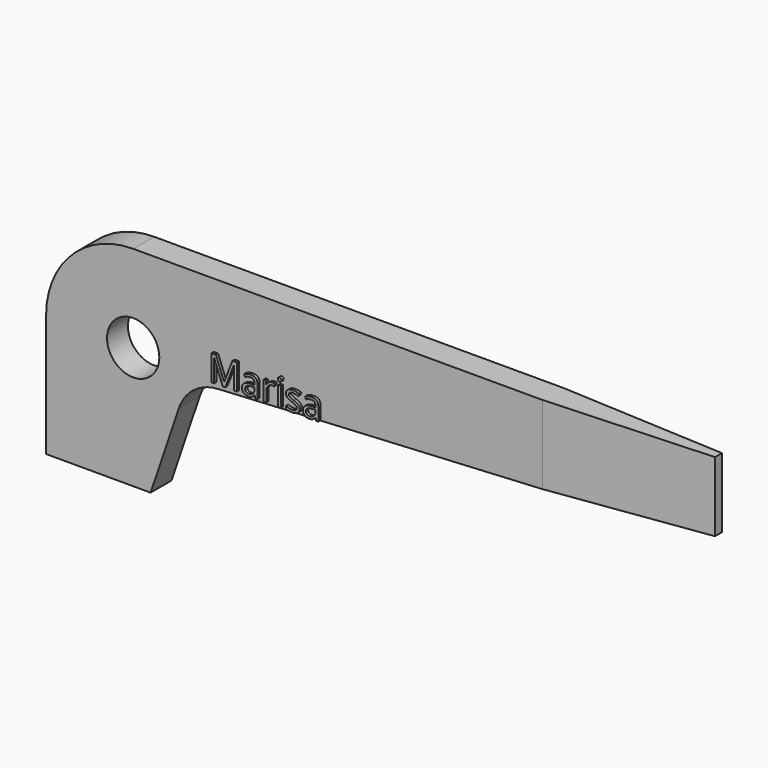
from build123d import *

# Parameters (mm, degrees)
F1_DEPTH     = 2.38125
F2_R         = 2.38125
F3_DEPTH     = 25.4
F5_DEPTH     = 25.4
F6_TEXT_SIZE = 3.2750783396
F7_DEPTH     = 0.254


# Not quite as in the source:
# - Text() gives the source's letters only with a copy of the font that has no kerning and outlines rounded to 1/6400 em; it was checked with that copy


with BuildPart() as f1:
    # F0 (on Front) → F1 (new body)
    with BuildSketch(Plane.XZ):
        with BuildLine():
            Line((60.325, 19.05), (7.9375, 19.05))
            ThreePointArc((7.9375, 19.05), (2.3248399243, 16.7251600757), (0, 11.1125))
            Line((0, 11.1125), (0, 0))
            Line((0, 0), (9.525, 0))
            Line((9.525, 0), (12.1103451907, 7.6262422093))
            ThreePointArc((12.1103451907, 7.6262422093), (13.4737562991, 9.5178776332), (15.6634210502, 10.3194652484))
            Line((15.6634210502, 10.3194652484), (60.325, 12.7))
            Line((60.325, 12.7), (60.325, 19.05))
        make_face()
    extrude(amount=F1_DEPTH)

    # F2 (on face) → F3 (cut)
    with BuildSketch(Plane.XZ.offset(2.38125)):
        with Locations((7.9375, 11.1125)):
            Circle(F2_R)
    extrude(amount=-F3_DEPTH, mode=Mode.SUBTRACT)

    # F4 (on face) → F5 (cut)
    with BuildSketch(Plane.XY.offset(19.05)):
        Polygon((60.325, -2.38125), (60.325, -1.5875), (45.24375, -2.38125), align=None)
        Polygon((60.325, 0), (45.24375, 0), (60.325, -0.79375), align=None)
    extrude(amount=-F5_DEPTH, mode=Mode.SUBTRACT)

    # F6 (on face) → F7 (join)
    with BuildSketch(Plane.XZ.offset(2.38125)):
        with Locations((14.9520464325, 10.8291972317)):
            Text('Marisa', F6_TEXT_SIZE, font='Open Sans', text_align=(TextAlign.LEFT, TextAlign.BOTTOM))
    extrude(amount=F7_DEPTH)


solid = f1.part
